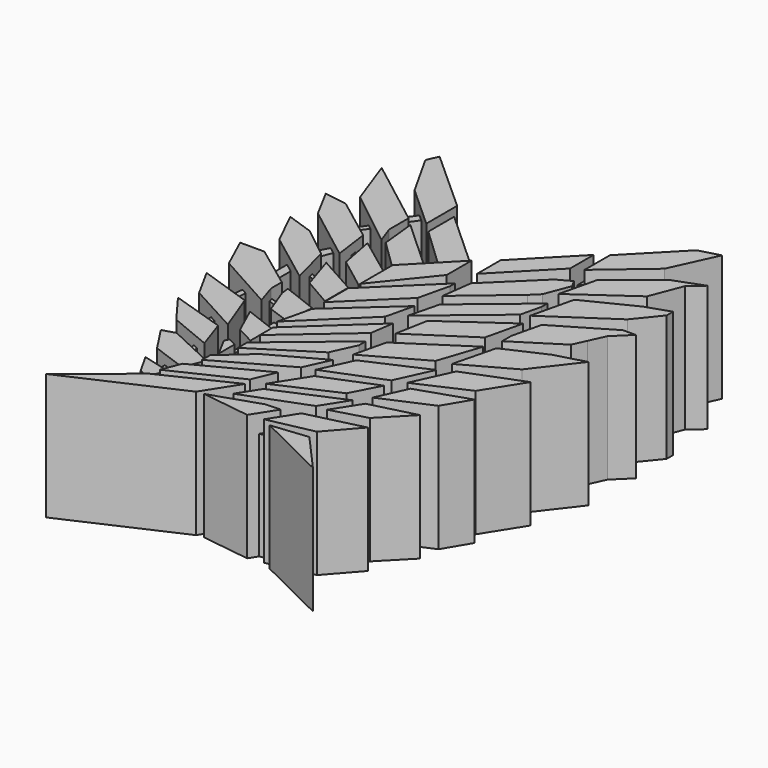
from build123d import *

# Parameters (mm, degrees)
F1_DEPTH = 29.718
F3_DEPTH = 25.4
F5_DEPTH = 2.032


# Not quite as in the source:
# - a feature names something its author has since deleted; it is built from what else it names


with BuildPart() as f1:
    # F0 (on Top) → F1 (new body)
    with BuildSketch(Plane.XY):
        Polygon((-25.1207519323, -10.9509155154), (-37.3962149024, -6.8106707186), (-33.5240279023, -13.8563495129), (-21.5468890965, -20.3935783356), align=None)
    extrude(amount=F1_DEPTH)



with BuildPart() as f1b:
    # F0 (on Top) → F1, piece 2 (new body)
    with BuildSketch(Plane.XY):
        Polygon((20.5661617219, -49.0451008081), (11.965691112, -49.9642342329), (28.762735726, -58.2453389419), align=None)
    extrude(amount=F1_DEPTH)


with BuildPart() as f1c:
    # F0 (on Top) → F1, piece 3 (new body)
    with BuildSketch(Plane.XY):
        Polygon((18.5046084225, 41.9357403646), (18.5046084225, 34.4622395933), (29.6869054437, 44.0044663846), (34.6125770394, 54.7369669283), (29.6869054437, 53.3975958824), align=None)
    extrude(amount=F1_DEPTH)


with BuildPart() as f1d:
    # F0 (on Top) → F1, piece 4 (new body)
    with BuildSketch(Plane.XY):
        Polygon((34.8864719272, 4.3231924064), (25.353750214, 0), (22.8669531643, -9.975887835), (34.2647694051, -3.6552799866), (41.9323928654, 6.291906815), align=None)
    extrude(amount=F1_DEPTH)


with BuildPart() as f1e:
    # F0 (on Top) → F1, piece 5 (new body)
    with BuildSketch(Plane.XY):
        Polygon((38.642052561, -6.6121835262), (25.353750214, -11.8024554104), (21.1496921354, -20.9626388974), (32.9574719071, -15.6333707273), align=None)
    extrude(amount=F1_DEPTH)


with BuildPart() as f1f:
    # F0 (on Top) → F1, piece 6 (new body)
    with BuildSketch(Plane.XY):
        Polygon((34.9347181618, -18.4756610543), (23.0712369084, -22.4301554263), (19.8582112789, -29.5395315605), (31.3509590924, -24.5309788734), align=None)
    extrude(amount=F1_DEPTH)


with BuildPart() as f1g:
    # F0 (on Top) → F1, piece 7 (new body)
    with BuildSketch(Plane.XY):
        Polygon((-1.8525850289, -39.9389926097), (-18.1308686733, -47.7529764175), (-32.8748077154, -59.6838273569), (-6.9757119046, -47.9948553431), align=None)
    extrude(amount=F1_DEPTH)


with BuildPart() as f1h:
    # F0 (on Top) → F1, piece 8 (new body)
    with BuildSketch(Plane.XY):
        Polygon((31.0155879706, -29.5395315605), (20.326230675, -32.2718434036), (16.3414671843, -38.537686215), (24.5036836714, -36.2035594881), align=None)
    extrude(amount=F1_DEPTH)


with BuildPart() as f1i:
    # F0 (on Top) → F1, piece 9 (new body)
    with BuildSketch(Plane.XY):
        Polygon((6.1410656199, -49.3182533124), (9.6368789673, -43.8212603331), (6.1410656199, -43.9441278577), (-5.2299234085, -47.7529764175), align=None)
    extrude(amount=F1_DEPTH)


with BuildPart() as f1j:
    # F0 (on Top) → F1, piece 10 (new body)
    with BuildSketch(Plane.XY):
        Polygon((26.5924073756, -39.3980778754), (13.5685950518, -42.5925962627), (9.6368789673, -48.7750246607), (20.326230675, -46.5243123472), align=None)
    extrude(amount=F1_DEPTH)


with BuildPart() as f1k:
    # F0 (on Top) → F1, piece 11 (new body)
    with BuildSketch(Plane.XY):
        Polygon((-32.8966340615, 56.0402274132), (-34.0748243034, 53.3613786101), (-28.118697453, 42.7545762411), (-18.1308686733, 33.7089374661), (-18.1308686733, 42.790748179), (-32.8512765426, 56.0402274132), align=None)
    extrude(amount=F1_DEPTH)


with BuildPart() as f1l:
    # F0 (on Top) → F1, piece 12 (new body)
    with BuildSketch(Plane.XY):
        Polygon((-22.7776132524, -8.9506592711), (-24.3092160672, -4.2026895098), (-24.3092160672, -1.05593975), (-34.4065353274, 6.4478195272), (-40.1176773012, 6.4478195272), (-36.6158593845, -1.2482392153), align=None)
    extrude(amount=F1_DEPTH)


with BuildPart() as f1m:
    # F0 (on Top) → F1, piece 13 (new body)
    with BuildSketch(Plane.XY):
        Polygon((-30.1326271147, -24.8243659735), (-20.254150033, -28.8919750601), (-22.6511321962, -21.8462962657), (-35.3624112904, -17.7786871791), align=None)
    extrude(amount=F1_DEPTH)


with BuildPart() as f1n:
    # F0 (on Top) → F1, piece 14 (new body)
    with BuildSketch(Plane.XY):
        Polygon((-20.254150033, -45.9143769149), (-18.7274646014, -41.7159944773), (-25.2524730425, -39.9735620477), (-22.6087478561, -44.6934739383), align=None)
    extrude(amount=F1_DEPTH)


with BuildPart() as f1o:
    # F0 (on Top) → F1, piece 15 (new body)
    with BuildSketch(Plane.XY):
        Polygon((4.0606590919, 20.9048669785), (16.0922389477, 33.2372374833), (16.0922389477, 40.1553977281), (4.0606590919, 27.8230272233), align=None)
    extrude(amount=F1_DEPTH)


with BuildPart() as f1p:
    # F0 (on Top) → F1, piece 16 (new body)
    with BuildSketch(Plane.XY):
        Polygon((32.9839587212, 40.987245331), (22.8388421237, 32.7328331769), (20.7784473896, 24.0064541903), (34.0493395925, 33.3972834051), (36.974107327, 40.987245331), (40.0701205218, 43.6291765906), align=None)
    extrude(amount=F1_DEPTH)


with BuildPart() as f1q:
    # F0 (on Top) → F1, piece 17 (new body)
    with BuildSketch(Plane.XY):
        Polygon((36.0025428236, 29.7452602535), (24.460894987, 24.0064541903), (22.0943034, 13.9832412824), (36.974107327, 24.0064541903), (41.6053501711, 29.7452602535), (41.6053501711, 31.621646136), align=None)
    extrude(amount=F1_DEPTH)


with BuildPart() as f1r:
    # F0 (on Top) → F1, piece 18 (new body)
    with BuildSketch(Plane.XY):
        Polygon((39.0159065823, 20.1370180575), (26.0368771851, 12.4609731138), (24.4053379095, 5.5509233966), (24.4053379095, 2.8386670165), (35.1527482271, 9.675568901), (36.5690001905, 12.7614272802), (38.2799704117, 16.4894445612), (42.0210714562, 20.1370180575), align=None)
    extrude(amount=F1_DEPTH)


with BuildPart() as f1s:
    # F0 (on Top) → F1, piece 19 (new body)
    with BuildSketch(Plane.XY):
        Polygon((-1.7404796529, 26.2233787644), (-15.8558022231, 39.0686951578), (-15.8558022231, 31.4757041633), (-5.7872179896, 21.9472479075), align=None)
    extrude(amount=F1_DEPTH)


with BuildPart() as f1t:
    # F0 (on Top) → F1, piece 20 (new body)
    with BuildSketch(Plane.XY):
        Polygon((-38.3924096823, 45.9172725677), (-34.2174710831, 34.3277863109), (-20.5516587645, 23.5672202222), (-22.014182061, 27.6271346956), (-22.014182061, 33.3647206426), align=None)
    extrude(amount=F1_DEPTH)


with BuildPart() as f1u:
    # F0 (on Top) → F1, piece 21 (new body)
    with BuildSketch(Plane.XY):
        Polygon((-23.1616999954, 14.4748231396), (-24.3092160672, 22.8605251759), (-34.7251407802, 30.7166036218), (-40.0213748217, 31.5110385418), (-36.2257398665, 24.4493950158), align=None)
    extrude(amount=F1_DEPTH)


with BuildPart() as f1v:
    # F0 (on Top) → F1, piece 22 (new body)
    with BuildSketch(Plane.XY):
        Polygon((-23.2947226614, 2.8717699461), (-25.7831495255, 12.3076587915), (-33.0430269241, 18.0707406253), (-39.3322594464, 20.2195607126), (-35.2790850681, 11.91082253), align=None)
    extrude(amount=F1_DEPTH)


with BuildPart() as f1w:
    # F0 (on Top) → F1, piece 23 (new body)
    with BuildSketch(Plane.XY):
        Polygon((-17.5666213036, -38.8837116485), (-15.6054534018, -34.1208763421), (-26.7923828214, -28.8919750601), (-29.7848970942, -29.7984248721), (-25.804895776, -35.8879736934), align=None)
    extrude(amount=F1_DEPTH)


with BuildPart() as f1x:
    # F0 (on Top) → F1, piece 24 (new body)
    with BuildSketch(Plane.XY):
        Polygon((0, -32.5635410845), (-15.8558022231, -40.8432632685), (-17.5858922303, -45.2920682728), (-2.2622323595, -38.0009710789), align=None)
    extrude(amount=F1_DEPTH)


with BuildPart() as f1y:
    # F0 (on Top) → F1, piece 25 (new body)
    with BuildSketch(Plane.XY):
        Polygon((-12.6461180425, 14.164019376), (-21.7168368399, 20.9048669785), (-20.1256703585, 12.572853826), (-12.6461180425, 6.9314968314), align=None)
    extrude(amount=F1_DEPTH)


with BuildPart() as f1z:
    # F0 (on Top) → F1, piece 26 (new body)
    with BuildSketch(Plane.XY):
        Polygon((-13.4074138477, 4.8822183162), (-22.7776132524, 10.0977066904), (-20.1256703585, 1.8766819267), (-13.4074138477, -2.0128341857), align=None)
    extrude(amount=F1_DEPTH)


with BuildPart() as f1ba:
    # F0 (on Top) → F1, piece 27 (new body)
    with BuildSketch(Plane.XY):
        Polygon((-21.8242239207, -2.3809622508), (-21.5468890965, -4.4147567824), (-19.2357581109, -10.6085864827), (-14.1512714326, -12.45749183), (-13.5041549802, -5.6165447459), align=None)
    extrude(amount=F1_DEPTH)


with BuildPart() as f1bb:
    # F0 (on Top) → F1, piece 28 (new body)
    with BuildSketch(Plane.XY):
        Polygon((-10.2059470555, 4.4086207636), (0, 17.0553233474), (0, 24.3715960532), (-10.2059470555, 13.9104993437), align=None)
    extrude(amount=F1_DEPTH)


with BuildPart() as f1bc:
    # F0 (on Top) → F1, piece 29 (new body)
    with BuildSketch(Plane.XY):
        Polygon((1.5137576265, 6.5658204257), (3.2650928479, 13.9832412824), (3.2650928479, 15.3817338329), (-10.8486106619, 1.620872994), (-10.8486106619, -5.4874885827), align=None)
    extrude(amount=F1_DEPTH)


with BuildPart() as f1bd:
    # F0 (on Top) → F1, piece 30 (new body)
    with BuildSketch(Plane.XY):
        Polygon((21.5263398801, 19.7248701006), (6.3493880443, 7.1178409271), (4.5737489127, 0), (20.3769281507, 13.1550095975), (21.5263398801, 18.0231070532), align=None)
    extrude(amount=F1_DEPTH)


with BuildPart() as f1be:
    # F0 (on Top) → F1, piece 31 (new body)
    with BuildSketch(Plane.XY):
        Polygon((8.647499606, 0.6018792628), (7.2285784408, -7.0254327729), (20.9934078157, 2.0141589921), (23.0558932898, 10.7493928786), align=None)
    extrude(amount=F1_DEPTH)


with BuildPart() as f1bf:
    # F0 (on Top) → F1, piece 32 (new body)
    with BuildSketch(Plane.XY):
        Polygon((4.352341406, -4.1491989978), (-11.8778329343, -19.1467050463), (-11.8778329343, -23.0501648039), (3.5305602942, -9.6962219104), align=None)
    extrude(amount=F1_DEPTH)


with BuildPart() as f1bg:
    # F0 (on Top) → F1, piece 33 (new body)
    with BuildSketch(Plane.XY):
        Polygon((-12.7423045157, -16.8832521719), (1.520585404, -2.9769345841), (3.0911655602, 3.6749352952), (-10.8486106619, -8.8629005477), align=None)
    extrude(amount=F1_DEPTH)


with BuildPart() as f1bh:
    # F0 (on Top) → F1, piece 34 (new body)
    with BuildSketch(Plane.XY):
        Polygon((23.0558932898, -1.0648668977), (8.1534059718, -10.8048198745), (6.3565219977, -18.4151531244), (19.7584591806, -10.9084369615), align=None)
    extrude(amount=F1_DEPTH)


with BuildPart() as f1bi:
    # F0 (on Top) → F1, piece 35 (new body)
    with BuildSketch(Plane.XY):
        Polygon((4.8764669239, -12.8880226985), (-11.8622847404, -26.8218290218), (-11.839268415, -29.5395315605), (2.2494671232, -20.5770652821), (4.8764669239, -14.8531195741), align=None)
    extrude(amount=F1_DEPTH)


with BuildPart() as f1bj:
    # F0 (on Top) → F1, piece 36 (new body)
    with BuildSketch(Plane.XY):
        Polygon((22.1077466219, -13.6575122529), (8.241889067, -19.8350194842), (4.7606257778, -27.4203120514), (18.2516984642, -22.0594201237), align=None)
    extrude(amount=F1_DEPTH)


with BuildPart() as f1bk:
    # F0 (on Top) → F1, piece 37 (new body)
    with BuildSketch(Plane.XY):
        Polygon((-14.0021331608, -35.0350998342), (-14.0021331608, -37.3830795288), (2.0629931241, -28.3618941903), (4.8100714807, -22.3763104211), (-7.2053484619, -28.9797838777), align=None)
    extrude(amount=F1_DEPTH)


with BuildPart() as f1bl:
    # F0 (on Top) → F1, piece 38 (new body)
    with BuildSketch(Plane.XY):
        Polygon((18.4988547117, -24.5309788734), (6.1410656199, -29.5395315605), (1.0743702296, -37.5066585839), (15.0386719033, -31.2041863799), align=None)
    extrude(amount=F1_DEPTH)


with BuildPart() as f1bm:
    # F0 (on Top) → F1, piece 39 (new body)
    with BuildSketch(Plane.XY):
        Polygon((19.7482518852, 29.7452602535), (16.554640606, 27.9939249158), (5.5535457381, 17.2678574843), (4.6043489128, 10.0684920326), (16.554640606, 20.1644264162), (18.4876212478, 22.0490825305), (20.7784473896, 27.9939249158), align=None)
    extrude(amount=F1_DEPTH)


with BuildPart() as f1bn:
    # F0 (on Top) → F1, piece 40 (new body)
    with BuildSketch(Plane.XY):
        Polygon((-15.6054534018, -25.8412677795), (-17.5666213036, -24.8243659735), (-18.1064039113, -25.865375359), (-15.6054534018, -30.4899644107), align=None)
    extrude(amount=F1_DEPTH)


with BuildPart() as f1bo:
    # F0 (on Top) → F1, piece 41 (new body)
    with BuildSketch(Plane.XY):
        Polygon((-7.7226855792, 20.1606620103), (-20.0799051672, 31.4757041633), (-19.2104098591, 23.1325210437), (-11.839268415, 15.9411642093), align=None)
    extrude(amount=F1_DEPTH)


with BuildPart() as f1bp:
    # F0 (on Top) → F1, piece 42 (new body)
    with BuildSketch(Plane.XY):
        Polygon((17.6019282588, -32.7050656735), (2.0191774238, -39.3980778754), (-1.1110491361, -44.3202037768), (13.814327307, -38.6608801782), align=None)
    extrude(amount=F1_DEPTH)


with BuildPart() as f1bq:
    # F0 (on Top) → F1, piece 43 (new body)
    with BuildSketch(Plane.XY):
        Polygon((-14.2980078235, -16.61651209), (-21.5468890965, -13.8563495129), (-18.4800280657, -20.6515516557), (-14.2980078235, -22.7905623615), align=None)
    extrude(amount=F1_DEPTH)


with BuildPart() as f1_1:
    add(f1.part)

    add(f1b.part)  # F3 merges F1b

    add(f1c.part)  # F3 merges F1c

    add(f1d.part)  # F3 merges F1d

    add(f1e.part)  # F3 merges F1e

    add(f1f.part)  # F3 merges F1f

    add(f1g.part)  # F3 merges F1g

    add(f1h.part)  # F3 merges F1h

    add(f1i.part)  # F3 merges F1i

    add(f1j.part)  # F3 merges F1j

    add(f1k.part)  # F3 merges F1k

    add(f1l.part)  # F3 merges F1l

    add(f1m.part)  # F3 merges F1m

    add(f1n.part)  # F3 merges F1n

    add(f1o.part)  # F3 merges F1o

    add(f1p.part)  # F3 merges F1p

    add(f1q.part)  # F3 merges F1q

    add(f1r.part)  # F3 merges F1r

    add(f1s.part)  # F3 merges F1s

    add(f1t.part)  # F3 merges F1t

    add(f1u.part)  # F3 merges F1u

    add(f1v.part)  # F3 merges F1v

    add(f1w.part)  # F3 merges F1w

    add(f1x.part)  # F3 merges F1x

    add(f1y.part)  # F3 merges F1y

    add(f1z.part)  # F3 merges F1z

    add(f1ba.part)  # F3 merges F1ba

    add(f1bb.part)  # F3 merges F1bb

    add(f1bc.part)  # F3 merges F1bc

    add(f1bd.part)  # F3 merges F1bd

    add(f1be.part)  # F3 merges F1be

    add(f1bf.part)  # F3 merges F1bf

    add(f1bg.part)  # F3 merges F1bg

    add(f1bh.part)  # F3 merges F1bh

    add(f1bi.part)  # F3 merges F1bi

    add(f1bj.part)  # F3 merges F1bj

    add(f1bk.part)  # F3 merges F1bk

    add(f1bl.part)  # F3 merges F1bl

    add(f1bm.part)  # F3 merges F1bm

    add(f1bn.part)  # F3 merges F1bn

    add(f1bo.part)  # F3 merges F1bo

    add(f1bp.part)  # F3 merges F1bp

    add(f1bq.part)  # F3 merges F1bq
    # F2 (on Top) + F0 (on Top) → F3 (join)
    with BuildSketch(Plane.XY):
        Polygon((-16.8312812905, 26.064571603), (-23.088272661, 31.0089010745), (-23.5761385411, 29.7404490411), (-17.624175176, 25.0569358468), align=None)
        Polygon((-22.6774581196, 40.097479689), (-23.6290413886, 39.3243543804), (-26.9407853484, 34.6327200532), (-25.3155075279, 33.4854643999), (-21.3230575591, 39.1414316336), align=None)
        Polygon((-27.2224399486, 29.7140372861), (-28.017161414, 30.8445319533), (-31.3912531941, 26.064571603), (-30.3282153923, 25.3141915065), align=None)
        Polygon((-26.1196792126, 19.2500371486), (-27.7791395783, 19.97307688), (-30.6563749909, 14.5382992923), (-28.4971518306, 13.3951810616), align=None)
        Polygon((-28.4971518306, 8.9874407277), (-30.6563749909, 9.7478022799), (-30.6563749909, 1.7640031874), (-28.4971518306, 0), align=None)
        Polygon((-29.3305683881, -3.5373331048), (-30.6563749909, -3.0852193013), (-31.4781107008, -10.2060129866), (-29.9583806634, -10.7411796667), align=None)
        Polygon((-27.0588895507, -15.3189375997), (-28.4971518306, -15.3189375997), (-28.4971518306, -21.7820126563), (-27.0588895507, -21.9073566245), align=None)
        Polygon((-23.2096277177, -25.6825387478), (-24.2356862873, -26.2688584626), (-23.2096277177, -31.9854691625), (-22.0458292595, -32.0868937211), align=None)
        Polygon((-22.0458292595, -35.7372611761), (-23.2096277177, -36.1174419522), (-23.2096277177, -41.4399765432), (-22.0458292595, -41.5414011018), align=None)
        Polygon((-19.8144204915, 17.9872009903), (-24.7876737267, 20.5868557096), (-24.7876737267, 19.3435419351), (-19.8144204915, 16.7438872159), align=None)
        Polygon((-19.8144204915, 6.4439540729), (-25.7439650595, 8.7962038815), (-25.7439650595, 7.8236756337), (-20.1477638449, 5.6036631041), align=None)
        Polygon((-19.8144204915, -5.4784687236), (-25.7439650595, -3.4502635244), (-25.7439650595, -4.2794439942), (-19.8144204915, -6.6316938028), align=None)
        Polygon((-18.1557461619, -9.7460197285), (-18.1557461619, -16.1979049444), (-16.5874008089, -17.230771482), (-16.5874008089, -9.7460197285), align=None)
        Polygon((-14.3431518227, 11.8969893083), (-8.8542243466, 10.7316616923), (-9.0206200257, 11.8969893083), (-14.3431518227, 13.0375316367), align=None)
        Polygon((-14.378025292, 0), (-9.971071966, -1.7895249184), (-10.3587438467, 0), (-14.378025292, 1.6321035801), align=None)
        Polygon((-15.7724563032, -8.9675774798), (-10.3587438467, -11.752593331), (-10.3587438467, -10.8731146902), (-15.7724563032, -8.0880988389), align=None)
        Polygon((-16.9262010604, -19.9088156223), (-16.9262010604, -25.6115309894), (-16.2845477462, -26.3876691461), (-15.7724563032, -20.3773150231), align=None)
        Polygon((-12.3433154076, 19.1328395158), (-7.4009639211, 15.3310308233), (-6.070329342, 15.9013010561), (-11.8111973444, 20.4432540534), align=None)
        Polygon((-5.5560725741, 24.1229701787), (-2.4778975639, 20.4584766179), (-1.7449983861, 20.8982154727), (-5.4774540116, 25.0457065532), align=None)
        Polygon((-19.8144204915, 36.8371625411), (-14.4431963563, 34.6560776234), (-14.2326668675, 36.8594056832), (-19.3735323846, 38.3538305759), align=None)
        Polygon((5.1145781763, 26.064571603), (-0.9683163371, 19.0062150359), (-0.7782261819, 17.6755804569), (5.1145781763, 24.3287459016), align=None)
        Polygon((14.7023710988, 36.8594056832), (14.9204516783, 34.6560776234), (20.3552301973, 38.334723562), (19.2639302245, 39.9469944217), align=None)
        Polygon((22.9127705097, 40.8922657371), (27.38847211, 34.8181053996), (29.6936274617, 34.8181053996), (24.4067749835, 41.9931122479), align=None)
        Polygon((25.4703145474, 30.0227124244), (27.38847211, 24.5879348367), (29.9213718267, 24.2595467775), (27.38847211, 31.4360931051), align=None)
        Polygon((27.38847211, 19.7691134585), (29.9213718267, 12.5925671309), (31.4249639375, 12.5925671309), (28.5817401954, 20.6483645126), align=None)
        Polygon((28.5817401954, 8.0557973817), (31.4249639375, 0), (33.1129832326, 0), (29.9213718267, 9.0428953677), align=None)
        Polygon((28.5817401954, -4.238050431), (28.5817401954, -11.8416687474), (29.9213718267, -12.4119408429), (29.9213718267, -3.250952445), align=None)
        Polygon((27.38847211, -15.4237812385), (27.38847211, -22.5727688521), (28.5817401954, -22.8192862123), (28.5817401954, -15.5784873203), align=None)
        Polygon((19.9066214263, -36.0728874803), (17.815625295, -42.5359643996), (19.1462598741, -43.6765067279), (21.2152574398, -36.2425509051), align=None)
        Polygon((23.5771182925, -25.7539637387), (23.5771182925, -32.4071310461), (25.4703145474, -32.7873118222), (25.4703145474, -25.9994148475), align=None)
        Polygon((15.0251089521, -46.1155591159), (16.5588241071, -50.4610836506), (18.4037955429, -51.0715047384), (16.7327779522, -46.3369567911), align=None)
        Polygon((5.8120195754, -47.649461776), (12.8610702232, -46.3369567911), (13.58074788, -44.4247052073), (5.8120195754, -46.1155591159), align=None)
        Polygon((5.33473947, -39.5947227545), (3.2250564545, -46.1155591159), (4.2617621718, -47.0916111982), (6.632780142, -39.7630125033), align=None)
        Polygon((8.927769959, -31.2917903066), (8.927769959, -37.9449538887), (10.1857112908, -38.1350442767), (10.1857112908, -30.3648852334), align=None)
        Polygon((11.208855547, -22.5727688521), (11.208855547, -29.2007941753), (12.8610702232, -29.3908845633), (12.8610702232, -21.3553462852), align=None)
        Polygon((12.8610702232, -10.5545492843), (12.8610702232, -19.6756720543), (15.0251089521, -19.4291546941), (15.0251089521, -8.9599928247), align=None)
        Polygon((13.6307686662, 0), (15.0251089521, -7.4885622598), (16.5588241071, -7.209691091), (15.0251089521, 1.0274096669), align=None)
        Polygon((12.8610702232, 9.0014694523), (15.0251089521, 2.8700288385), (16.5588241071, 3.5492809064), (15.0251089521, 10.5960259119), align=None)
        Polygon((11.208855547, 17.9793805418), (12.8610702232, 10.3881824762), (14.3079785934, 11.4259142348), (12.8610702232, 19.1968031087), align=None)
        Polygon((9.5073131203, 28.3108342229), (11.8237258866, 21.7476673424), (12.8610702232, 22.4216233293), (10.5193355141, 29.0565356854), align=None)
        Polygon((-5.2032573149, 12.8819094971), (-3.1303053256, 6.6630556248), (-1.7816288164, 7.3692854494), (-4.3281779214, 13.8973179297), align=None)
        Polygon((-6.723980885, 1.0963003151), (-4.0627145208, -3.8460518699), (-3.1303053256, -3.6559617147), (-5.6868767898, 2.2997159727), align=None)
        Polygon((1.3975448674, 11.2682590261), (1.3975448674, 10.3178070858), (6.9101690315, 13.9295263216), (6.2219943118, 14.5225955703), align=None)
        Polygon((6.8716742098, 5.5586574599), (0, -0.7709367783), (0, -2.014249796), (6.8716742098, 3.7502020132), align=None)
        Polygon((2.1100281738, -7.4523556978), (2.5497674942, -8.4784142673), (10.5193355141, -3.8460518699), (9.9565503291, -2.2514944835), align=None)
        Polygon((-4.8772442879, -6.8920103333), (-3.1303053256, -11.8416687474), (-1.982193433, -11.8416687474), (-4.0627145208, -5.9468613556), align=None)
        Polygon((-5.409494219, -15.4237812385), (-4.0627145208, -21.6116402298), (-2.6607783519, -21.0822355821), (-4.0627145208, -14.6409569228), align=None)
        Polygon((-3.664197017, -23.1808127531), (-2.6316980366, -27.9246903956), (-1.5389597353, -27.5199755198), (-2.6316980366, -22.4993247539), align=None)
        Polygon((-6.0780528001, -30.8762919158), (-6.0780528001, -36.7158018053), (-5.3402668565, -36.8901155889), (-5.3402668565, -30.447449116), align=None)
        Polygon((-14.8724438623, -19.4291546941), (-14.6036148071, -20.2430319041), (-11.4448796958, -21.1839322001), (-11.4448796958, -20.5118618906), align=None)
        Polygon((-16.1774531007, -27.1609826612), (-16.1774531007, -27.9246903956), (-10.3587438467, -27.9246903956), (-10.8026538532, -27.1609826612), align=None)
        Polygon((-18.4380225837, -34.9778831005), (-18.3249935508, -36.2211987376), (-11.7693431675, -35.4299992323), (-11.9953993708, -34.4127416611), align=None)
        Polygon((-20.7567772354, -43.5170159414), (-20.5714888871, -44.315662235), (-14.971932834, -43.0969259287), (-15.2469178587, -42.3178020035), align=None)
        Polygon((-7.9465830192, -39.5605285169), (-7.1826991625, -43.0702380836), (-6.3590905557, -43.1678334767), (-7.2343236595, -39.1465232074), align=None)
        Polygon((-13.7194646522, -42.1115159988), (-13.7194646522, -46.5565137565), (-12.847895734, -46.817984432), (-12.847895734, -42.1115159988), align=None)
        Polygon((-7.1826991625, -45.9239073098), (-1.1412214953, -47.754202038), (0.7192745837, -47.0444114289), (-6.8293374516, -44.7575230921), align=None)
        Polygon((-5.0167776644, -43.4282831848), (2.5497674942, -42.1209298074), (2.5497674942, -41.2493608892), (-5.0167776644, -42.3824004829), align=None)
        Polygon((-3.0673491858, -35.4299992323), (-2.6316980366, -36.7158018053), (5.1145781763, -33.9818208722), (4.420262149, -32.7873118222), align=None)
        Polygon((11.208855547, -38.6521629989), (15.0251089521, -43.5329452157), (16.1012466997, -43.0702380836), (11.8183286412, -37.9449538887), align=None)
        Polygon((1.224700056, -25.617185331), (1.7104209401, -26.8279705197), (8.7437685579, -23.9766146988), (8.25363514, -22.7676183743), align=None)
        Polygon((1.0725045347, -17.4557565189), (1.7104209401, -19.023405388), (10.2213893594, -14.0763505448), (9.3791991636, -12.6274371232), align=None)
        Polygon((14.7841639933, -26.8279705197), (15.7919665296, -28.0466899276), (25.7212538272, -24.0547899157), (25.0177218253, -23.2161251348), align=None)
        Polygon((13.6223621666, -35.3608727455), (13.4480493143, -36.0728874803), (21.5427014456, -35.0959463093), (21.4082379762, -33.9818208722), align=None)
        Polygon((18.106771633, -17.980504781), (18.219800666, -19.3368457258), (24.7754491866, -17.6414195448), (24.6291711106, -16.4294016934), align=None)
        Polygon((19.9066214263, -4.9750233569), (19.9066214263, -6.7474604584), (26.1111574251, -4.557623348), (25.3923114602, -2.7695955699), align=None)
        Polygon((19.9080727015, 6.2534315612), (20.1690271497, 4.8360642977), (27.0582791418, 8.0557973817), (26.4678323331, 9.3191744217), align=None)
        Polygon((19.2871445976, 15.4581444056), (19.6725912392, 14.5857119933), (25.9478855878, 18.2463005185), (25.4703145474, 19.0649936959), align=None)
        Polygon((23.7622718373, 29.6008122326), (18.4671729803, 26.5120044351), (18.5864082387, 25.1768369147), (24.3736531953, 28.5527299492), align=None)
    with BuildSketch(Plane.XY):
        Polygon((4.0606590919, 20.9048669785), (16.0922389477, 33.2372374833), (16.0922389477, 40.1553977281), (4.0606590919, 27.8230272233), align=None)
        Polygon((18.5046084225, 41.9357403646), (18.5046084225, 34.4622395933), (29.6869054437, 44.0044663846), (34.6125770394, 54.7369669283), (29.6869054437, 53.3975958824), align=None)
        Polygon((-10.2059470555, 4.4086207636), (0, 17.0553233474), (0, 24.3715960532), (-10.2059470555, 13.9104993437), align=None)
        Polygon((1.5137576265, 6.5658204257), (3.2650928479, 13.9832412824), (3.2650928479, 15.3817338329), (-10.8486106619, 1.620872994), (-10.8486106619, -5.4874885827), align=None)
        Polygon((19.7482518852, 29.7452602535), (16.554640606, 27.9939249158), (5.5535457381, 17.2678574843), (4.6043489128, 10.0684920326), (16.554640606, 20.1644264162), (18.4876212478, 22.0490825305), (20.7784473896, 27.9939249158), align=None)
        Polygon((32.9839587212, 40.987245331), (22.8388421237, 32.7328331769), (20.7784473896, 24.0064541903), (34.0493395925, 33.3972834051), (36.974107327, 40.987245331), (40.0701205218, 43.6291765906), align=None)
        Polygon((36.0025428236, 29.7452602535), (24.460894987, 24.0064541903), (22.0943034, 13.9832412824), (36.974107327, 24.0064541903), (41.6053501711, 29.7452602535), (41.6053501711, 31.621646136), align=None)
        Polygon((21.5263398801, 19.7248701006), (6.3493880443, 7.1178409271), (4.5737489127, 0), (20.3769281507, 13.1550095975), (21.5263398801, 18.0231070532), align=None)
        Polygon((4.8764669239, -12.8880226985), (-11.8622847404, -26.8218290218), (-11.839268415, -29.5395315605), (2.2494671232, -20.5770652821), (4.8764669239, -14.8531195741), align=None)
        Polygon((4.352341406, -4.1491989978), (-11.8778329343, -19.1467050463), (-11.8778329343, -23.0501648039), (3.5305602942, -9.6962219104), align=None)
        Polygon((-12.7423045157, -16.8832521719), (1.520585404, -2.9769345841), (3.0911655602, 3.6749352952), (-10.8486106619, -8.8629005477), align=None)
        Polygon((8.647499606, 0.6018792628), (7.2285784408, -7.0254327729), (20.9934078157, 2.0141589921), (23.0558932898, 10.7493928786), align=None)
        Polygon((39.0159065823, 20.1370180575), (26.0368771851, 12.4609731138), (24.4053379095, 5.5509233966), (24.4053379095, 2.8386670165), (35.1527482271, 9.675568901), (36.5690001905, 12.7614272802), (38.2799704117, 16.4894445612), (42.0210714562, 20.1370180575), align=None)
        Polygon((34.8864719272, 4.3231924064), (25.353750214, 0), (22.8669531643, -9.975887835), (34.2647694051, -3.6552799866), (41.9323928654, 6.291906815), align=None)
        Polygon((23.0558932898, -1.0648668977), (8.1534059718, -10.8048198745), (6.3565219977, -18.4151531244), (19.7584591806, -10.9084369615), align=None)
        Polygon((-14.0021331608, -35.0350998342), (-14.0021331608, -37.3830795288), (2.0629931241, -28.3618941903), (4.8100714807, -22.3763104211), (-7.2053484619, -28.9797838777), align=None)
        Polygon((-1.8525850289, -39.9389926097), (-18.1308686733, -47.7529764175), (-32.8748077154, -59.6838273569), (-6.9757119046, -47.9948553431), align=None)
        Polygon((0, -32.5635410845), (-15.8558022231, -40.8432632685), (-17.5858922303, -45.2920682728), (-2.2622323595, -38.0009710789), align=None)
        Polygon((22.1077466219, -13.6575122529), (8.241889067, -19.8350194842), (4.7606257778, -27.4203120514), (18.2516984642, -22.0594201237), align=None)
        Polygon((38.642052561, -6.6121835262), (25.353750214, -11.8024554104), (21.1496921354, -20.9626388974), (32.9574719071, -15.6333707273), align=None)
        Polygon((18.4988547117, -24.5309788734), (6.1410656199, -29.5395315605), (1.0743702296, -37.5066585839), (15.0386719033, -31.2041863799), align=None)
        Polygon((34.9347181618, -18.4756610543), (23.0712369084, -22.4301554263), (19.8582112789, -29.5395315605), (31.3509590924, -24.5309788734), align=None)
        Polygon((17.6019282588, -32.7050656735), (2.0191774238, -39.3980778754), (-1.1110491361, -44.3202037768), (13.814327307, -38.6608801782), align=None)
        Polygon((31.0155879706, -29.5395315605), (20.326230675, -32.2718434036), (16.3414671843, -38.537686215), (24.5036836714, -36.2035594881), align=None)
        Polygon((6.1410656199, -49.3182533124), (9.6368789673, -43.8212603331), (6.1410656199, -43.9441278577), (-5.2299234085, -47.7529764175), align=None)
        Polygon((26.5924073756, -39.3980778754), (13.5685950518, -42.5925962627), (9.6368789673, -48.7750246607), (20.326230675, -46.5243123472), align=None)
        Polygon((-32.8966340615, 56.0402274132), (-34.0748243034, 53.3613786101), (-28.118697453, 42.7545762411), (-18.1308686733, 33.7089374661), (-18.1308686733, 42.790748179), (-32.8512765426, 56.0402274132), align=None)
        Polygon((-32.8837707639, 56.0694746673), (-32.8966340615, 56.0402274132), (-32.8512765426, 56.0402274132), align=None)
        Polygon((-1.7404796529, 26.2233787644), (-15.8558022231, 39.0686951578), (-15.8558022231, 31.4757041633), (-5.7872179896, 21.9472479075), align=None)
        Polygon((-7.7226855792, 20.1606620103), (-20.0799051672, 31.4757041633), (-19.2104098591, 23.1325210437), (-11.839268415, 15.9411642093), align=None)
        Polygon((-38.3924096823, 45.9172725677), (-34.2174710831, 34.3277863109), (-20.5516587645, 23.5672202222), (-22.014182061, 27.6271346956), (-22.014182061, 33.3647206426), align=None)
        Polygon((-23.1616999954, 14.4748231396), (-24.3092160672, 22.8605251759), (-34.7251407802, 30.7166036218), (-40.0213748217, 31.5110385418), (-36.2257398665, 24.4493950158), align=None)
        Polygon((-12.6461180425, 14.164019376), (-21.7168368399, 20.9048669785), (-20.1256703585, 12.572853826), (-12.6461180425, 6.9314968314), align=None)
        Polygon((-13.4074138477, 4.8822183162), (-22.7776132524, 10.0977066904), (-20.1256703585, 1.8766819267), (-13.4074138477, -2.0128341857), align=None)
        Polygon((-23.2947226614, 2.8717699461), (-25.7831495255, 12.3076587915), (-33.0430269241, 18.0707406253), (-39.3322594464, 20.2195607126), (-35.2790850681, 11.91082253), align=None)
        Polygon((-22.7776132524, -8.9506592711), (-24.3092160672, -4.2026895098), (-24.3092160672, -1.05593975), (-34.4065353274, 6.4478195272), (-40.1176773012, 6.4478195272), (-36.6158593845, -1.2482392153), align=None)
        Polygon((-21.8242239207, -2.3809622508), (-21.5468890965, -4.4147567824), (-19.2357581109, -10.6085864827), (-14.1512714326, -12.45749183), (-13.5041549802, -5.6165447459), align=None)
        Polygon((-14.2980078235, -16.61651209), (-21.5468890965, -13.8563495129), (-18.4800280657, -20.6515516557), (-14.2980078235, -22.7905623615), align=None)
        Polygon((-25.1207519323, -10.9509155154), (-37.3962149024, -6.8106707186), (-33.5240279023, -13.8563495129), (-21.5468890965, -20.3935783356), align=None)
        Polygon((-15.6054534018, -25.8412677795), (-17.5666213036, -24.8243659735), (-18.1064039113, -25.865375359), (-15.6054534018, -30.4899644107), align=None)
        Polygon((-30.1326271147, -24.8243659735), (-20.254150033, -28.8919750601), (-22.6511321962, -21.8462962657), (-35.3624112904, -17.7786871791), align=None)
        Polygon((-17.5666213036, -38.8837116485), (-15.6054534018, -34.1208763421), (-26.7923828214, -28.8919750601), (-29.7848970942, -29.7984248721), (-25.804895776, -35.8879736934), align=None)
        Polygon((-20.254150033, -45.9143769149), (-18.7274646014, -41.7159944773), (-25.2524730425, -39.9735620477), (-22.6087478561, -44.6934739383), align=None)
        Polygon((20.5661617219, -49.0451008081), (11.965691112, -49.9642342329), (28.762735726, -58.2453389419), align=None)
    extrude(amount=F3_DEPTH)

    # F4 (on face) → F5 (cut)
    with BuildSketch(Plane.XY.offset(29.718)):
        Polygon((2.4770256249, 28.1880547751), (-34.5635004342, 61.5273267031), (-67.6095038652, 42.7545762411), (-37.4172367156, -47.8118807077), (-18.7672384929, -46.615484717), (-16.0798378731, -39.4490787586), (-13.412813656, -32.3370099068), (-13.412813656, -14.1145205125), (-12.0516363531, 1.419326989), (-11.3734658808, 3.2277826685), (-11.3734658808, 14.1915436834), (-10.4692382738, 15.2088003233), align=None)
    extrude(amount=-F5_DEPTH, mode=Mode.SUBTRACT)


solid = f1_1.part
